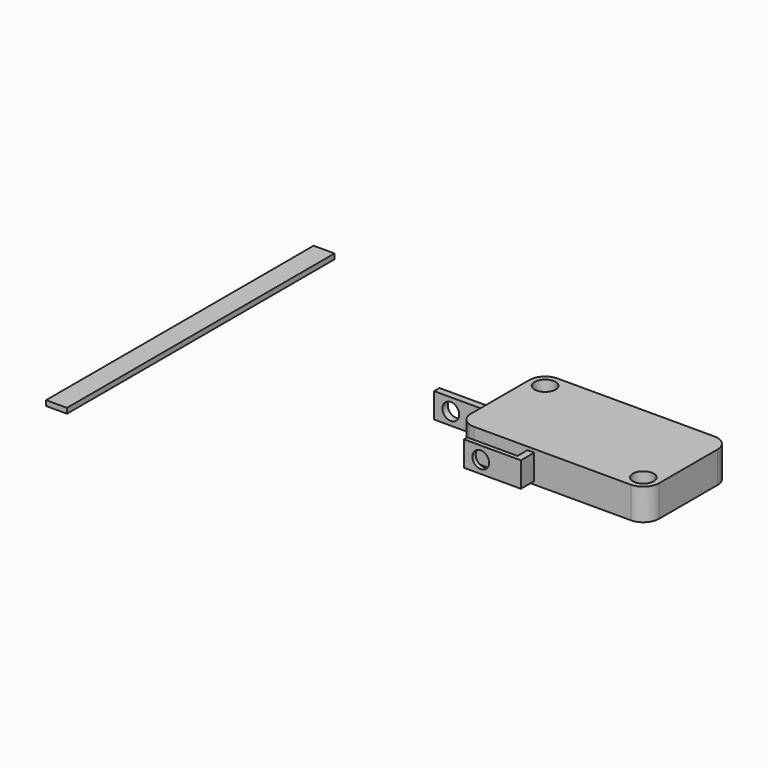
from build123d import *

# Parameters (mm, degrees)
F0_R      = 1.5875
F1_DEPTH  = 4.7625
F2_W      = 3.175
F2_H      = 50.8
F3_DEPTH  = 0.79375
F4_W      = 0.79375
F4_H      = 3.175
F5_DEPTH  = 0.79375
F6_W      = 1.016
F6_H      = 3.81
F7_DEPTH  = 2.54
F8_W      = 0.635
F8_H      = 3.81
F9_DEPTH  = 7.62
F10_R     = 1.27
F11_DEPTH = 1.16693
F12_W     = 1.016
F12_H     = 3.81
F13_DEPTH = 7.62
F14_R     = 1.27
F15_DEPTH = 25.4


# Not quite as in the source:
# - a length typed as a fraction of an inch, garbled in the dataset ("3 / 203.2 mm" for 3/8 in), is restored


with BuildPart() as f1:
    # F0 (on Top) → F1 (new body)
    with BuildSketch(Plane.XY):
        with BuildLine():
            ThreePointArc((7.3293575469, 20.2963850541), (6.6319055696, 21.9801830768), (4.9481075469, 22.6776350541))
            ThreePointArc((4.9481075469, 22.6776350541), (3.2643095242, 18.6125870314), (7.3293575469, 20.2963850541))
        make_face()
        with BuildLine():
            ThreePointArc((-16.4831424531, 9.1838850541), (-18.8643924531, 11.5651350541), (-21.2456424531, 9.1838850541))
            ThreePointArc((-21.2456424531, 9.1838850541), (-20.5481904758, 7.5000870314), (-18.8643924531, 6.8026350541))
            ThreePointArc((-18.8643924531, 6.8026350541), (-17.1805944304, 7.5000870314), (-16.4831424531, 9.1838850541))
        make_face()
        with BuildLine():
            ThreePointArc((-16.4831424531, 20.2963850541), (-17.1805944304, 21.9801830768), (-18.8643924531, 22.6776350541))
            ThreePointArc((-18.8643924531, 22.6776350541), (-20.5481904758, 21.9801830768), (-21.2456424531, 20.2963850541))
            ThreePointArc((-21.2456424531, 20.2963850541), (-18.8643924531, 17.9151350541), (-16.4831424531, 20.2963850541))
        make_face()
        with Locations((-18.8643924531, 20.2963850541)):
            Circle(F0_R, mode=Mode.SUBTRACT)
        with BuildLine():
            ThreePointArc((4.9481075338, 6.8026350541), (6.631905565, 7.5000870268), (7.3293575469, 9.1838850541))
            ThreePointArc((7.3293575469, 9.1838850541), (3.2643095288, 10.8676830814), (4.9481075338, 6.8026350541))
        make_face()
        with Locations((4.9481075469, 9.1838850541)):
            Circle(F0_R, mode=Mode.SUBTRACT)
        with BuildLine():
            Line((4.9481075469, 22.6776350541), (-18.8643924531, 22.6776350541))
            ThreePointArc((-18.8643924531, 22.6776350541), (-17.1805944304, 21.9801830768), (-16.4831424531, 20.2963850541))
            ThreePointArc((-16.4831424531, 20.2963850541), (-18.8643924531, 17.9151350541), (-21.2456424531, 20.2963850541))
            Line((-21.2456424531, 20.2963850541), (-21.2456424531, 9.1838850541))
            ThreePointArc((-21.2456424531, 9.1838850541), (-18.8643924531, 11.5651350541), (-16.4831424531, 9.1838850541))
            ThreePointArc((-16.4831424531, 9.1838850541), (-17.1805944304, 7.5000870314), (-18.8643924531, 6.8026350541))
            Line((-18.8643924531, 6.8026350541), (4.9481075338, 6.8026350541))
            ThreePointArc((4.9481075338, 6.8026350541), (3.2643095288, 10.8676830814), (7.3293575469, 9.1838850541))
            Line((7.3293575469, 9.1838850541), (7.3293575469, 20.2963850541))
            ThreePointArc((7.3293575469, 20.2963850541), (3.2643095242, 18.6125870314), (4.9481075469, 22.6776350541))
        make_face()
    extrude(amount=F1_DEPTH)

    # F4 (on face) → F5 (join)
    with BuildSketch(Plane(origin=(0, 22.6776350541, 0), x_dir=(-1, 0, 0), z_dir=(0, 1, 0))):
        with Locations((5.7675174531, 2.3495)):
            Rectangle(F4_W, F4_H)
    extrude(amount=F5_DEPTH)

    # F6 (on face) → F7 (join)
    with BuildSketch(Plane.XZ.offset(-6.8026350541)):
        with Locations((-10.2283924531, 2.3749)):
            Rectangle(F6_W, F6_H)
    extrude(amount=F7_DEPTH)

    # F8 (on face) → F9 (join)
    with BuildSketch(Plane(origin=(-10.7363924531, 0, 0), x_dir=(0, -1, 0), z_dir=(-1, 0, 0))):
        with Locations((-4.5801350541, 2.3749)):
            Rectangle(F8_W, F8_H)
    extrude(amount=F9_DEPTH)

    # F10 (on face) → F11 (cut)
    with BuildSketch(Plane.XZ.offset(-4.2626350541)):
        with Locations((-15.8163924531, 2.3749)):
            Circle(F10_R)
    extrude(amount=-F11_DEPTH, mode=Mode.SUBTRACT)

    # F12 (on face) → F13 (join)
    with BuildSketch(Plane(origin=(-21.2456424531, 0, 0), x_dir=(0, -1, 0), z_dir=(-1, 0, 0))):
        with Locations((-12.2318850541, 2.3749)):
            Rectangle(F12_W, F12_H)
    extrude(amount=F13_DEPTH)

    # F14 (on face) → F15 (cut)
    with BuildSketch(Plane(origin=(0, 12.7398850541, 0), x_dir=(-1, 0, 0), z_dir=(0, 1, 0))):
        with Locations((26.3256424531, 2.3749)):
            Circle(F14_R)
    extrude(amount=-F15_DEPTH, mode=Mode.SUBTRACT)


with BuildPart() as f3:
    # F2 (on Top) → F3 (new body)
    with BuildSketch(Plane.XY):
        with Locations((-65.9492532059, 11.7886504158)):
            Rectangle(F2_W, F2_H)
    extrude(amount=F3_DEPTH)


solid = Compound([f1.part, f3.part])
